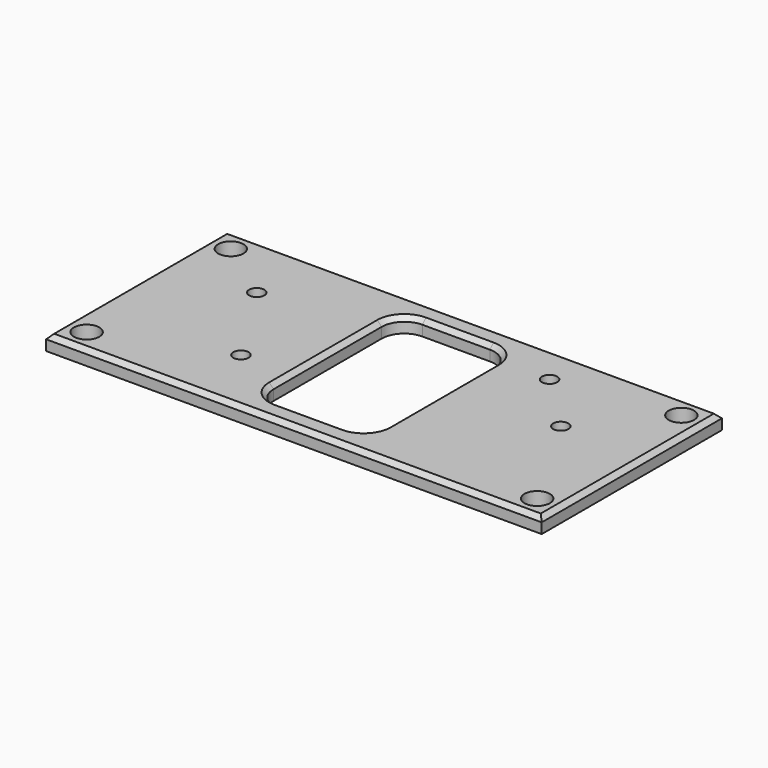
from build123d import *

# Parameters (mm, degrees)
F0_W           = 220
F0_H           = 100
F0_R           = 0.625
F0_W_2         = 50
F0_H_2         = 80
F0_R_2         = 0.6265
F1_DEPTH       = 6.6
F2_SIZE2       = 2
F2_SIZE        = 2
F3_D           = 6.8
F4_D           = 6.6
F4_CBORE_D     = 11.25
F4_CBORE_DEPTH = 6
F5_R           = 10
F6_SIZE2       = 2
F6_SIZE        = 2


# Not quite as in the source:
# - a feature names something its author has since deleted; it is built from what else it names


with BuildPart() as f1:
    # F0 (on Top) → F1 (new body)
    with BuildSketch(Plane.XY):
        with Locations((-110, -50)):
            Rectangle(F0_W, F0_H)
        with Locations((-157.5, -70)):
            Circle(F0_R, mode=Mode.SUBTRACT)
        with Locations((-182.5, -30)):
            Circle(F0_R, mode=Mode.SUBTRACT)
        with Locations((-110, -50)):
            Rectangle(F0_W_2, F0_H_2, mode=Mode.SUBTRACT)
        with Locations((-37.5, -42.5)):
            Circle(F0_R_2, mode=Mode.SUBTRACT)
        with Locations((-62.5, -17.5)):
            Circle(F0_R, mode=Mode.SUBTRACT)
    extrude(amount=-F1_DEPTH)

    # F2
    f2_edges = [f1.edges().sort_by_distance(p)[0] for p in [
        (-110, -100, 0),
        (0, -50, 0),
        (-110, 0, 0),
        (-220, -50, 0),
    ]]
    chamfer(f2_edges, length=F2_SIZE, length2=F2_SIZE2)

    # F3 (through all)
    with Locations(Plane.XY):
        with Locations((-182.5, -30), (-157.5, -70), (-37.5, -42.5), (-62.5, -17.5)):
            Hole(F3_D / 2)

    # F4 (through all)
    with Locations(Plane.XY):
        with Locations((-210, -10), (-210, -90), (-10, -90), (-10, -10)):
            CounterBoreHole(F4_D / 2, F4_CBORE_D / 2, F4_CBORE_DEPTH)

    # F5
    f5_edges = [f1.edges().sort_by_distance(p)[0] for p in [
        (-135, -10, -3.3),
        (-85, -10, -3.3),
        (-135, -90, -3.3),
        (-85, -90, -3.3),
    ]]
    fillet(f5_edges, radius=F5_R)

    # F6
    f6_edges = [f1.edges().sort_by_distance(p)[0] for p in [
        (-135, -50, 0),
    ]]
    chamfer(f6_edges, length=F6_SIZE, length2=F6_SIZE2)


solid = f1.part
